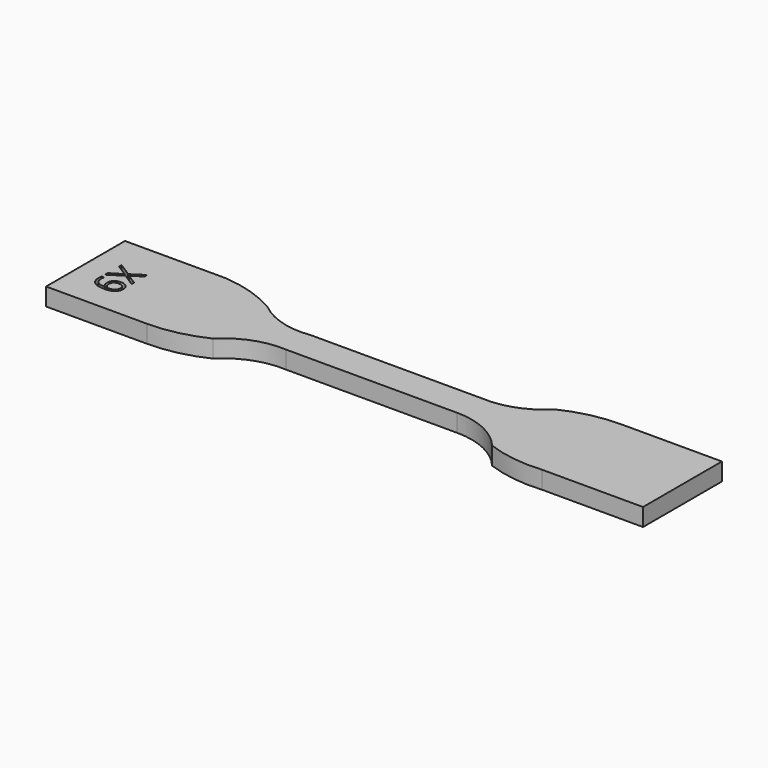
from build123d import *

# Parameters (mm, degrees)
F1_DEPTH     = 3.4
F2_TEXT_SIZE = 7.0564552314
F3_DEPTH     = 1


# Not quite as in the source:
# - Text() gives the source's letters only with a copy of the font that has no kerning and outlines rounded to 1/6400 em; it was checked with that copy


with BuildPart() as f1:
    # F0 (on Top) → F1 (new body)
    with BuildSketch(Plane.XY):
        with BuildLine():
            Line((-14.4320548165, 19.7811394548), (-33.8720548165, 19.7811394548))
            Line((-33.8720548165, 19.7811394548), (-33.8720548165, 0.7811394548))
            Line((-33.8720548165, 0.7811394548), (-14.4320548165, 0.7811394548))
            ThreePointArc((-14.4320548165, 0.7811394548), (-8.9053122052, 1.3996892086), (-3.6520548165, 3.2247301661))
            ThreePointArc((-3.6520548165, 3.2247301661), (1.3014698263, 6.4128780055), (7.1279451835, 7.2811394548))
            Line((7.1279451835, 7.2811394548), (40.1279451835, 7.2811394548))
            ThreePointArc((40.1279451835, 7.2811394548), (46.0837574042, 5.9511158081), (50.9079451835, 2.2137538538))
            ThreePointArc((50.9079451835, 2.2137538538), (56.2191047011, 0.9041953221), (61.6879451835, 0.7811394548))
            Line((61.6879451835, 0.7811394548), (81.1279451835, 0.7811394548))
            Line((81.1279451835, 0.7811394548), (81.1279451835, 19.7811394548))
            Line((81.1279451835, 19.7811394548), (61.6879451835, 19.7811394548))
            ThreePointArc((61.6879451835, 19.7811394548), (56.1612025723, 19.162589701), (50.9079451835, 17.3375487435))
            ThreePointArc((50.9079451835, 17.3375487435), (45.9544205407, 14.1494009041), (40.1279451835, 13.2811394548))
            Line((40.1279451835, 13.2811394548), (7.1279451835, 13.2811394548))
            ThreePointArc((7.1279451835, 13.2811394548), (1.4167452884, 13.6925537245), (-3.6520548165, 16.3560723447))
            ThreePointArc((-3.6520548165, 16.3560723447), (-8.8458057958, 18.686276846), (-14.4320548165, 19.7811394548))
        make_face()
    extrude(amount=F1_DEPTH)

    # F2 (on face) → F3 (cut)
    with BuildSketch(Plane.XY.offset(3.4)):
        with Locations(Location((-29.3720550835, 13.353464842), (0, 0, -90))):
            Text('X9', F2_TEXT_SIZE, font='Open Sans', text_align=(TextAlign.LEFT, TextAlign.BOTTOM))
    extrude(amount=-F3_DEPTH, mode=Mode.SUBTRACT)


solid = f1.part
